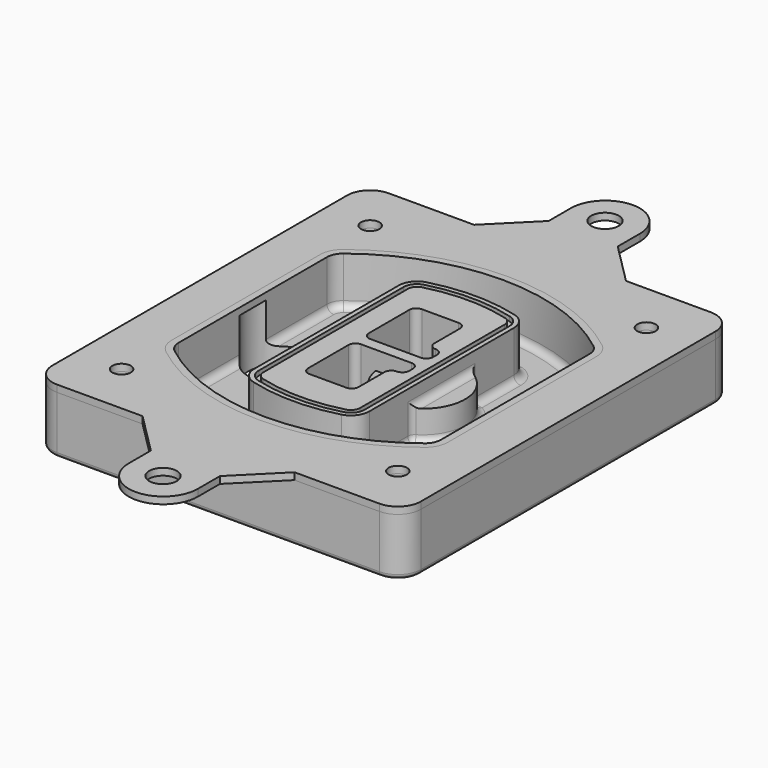
from build123d import *

# Parameters (mm, degrees)
F0_R      = 4
F1_DEPTH  = 25
F2_DEPTH  = 3
F3_DEPTH  = 18
F5_DEPTH  = 21
F6_DEPTH  = 2
F8_DEPTH  = 20
F9_DEPTH  = 16
F10_DEPTH = 25
F7_R      = 6
F7_R_2    = 4
F11_DEPTH = 6
F13_DEPTH = 9
F14_R     = 3
F15_R     = 2
F16_R     = 6
F16_R_2   = 4
F17_DEPTH = 3


with BuildPart() as f1:
    # F0 (on Top) → F1 (new body)
    with BuildSketch(Plane.XY):
        with BuildLine():
            ThreePointArc((-80, -80), (-77.0710678119, -87.0710678119), (-70, -90))
            Line((-70, -90), (70, -90))
            ThreePointArc((70, -90), (77.0710678119, -87.0710678119), (80, -80))
            Line((80, -80), (80, 80))
            ThreePointArc((80, 80), (77.0710678119, 87.0710678119), (70, 90))
            Line((70, 90), (-70, 90))
            ThreePointArc((-70, 90), (-77.0710678119, 87.0710678119), (-80, 80))
            Line((-80, 80), (-80, -80))
        make_face()
        with Locations((-60, -67.5)):
            Circle(F0_R, mode=Mode.SUBTRACT)
        with Locations((60, -67.5)):
            Circle(F0_R, mode=Mode.SUBTRACT)
        with Locations((-60, 67.5)):
            Circle(F0_R, mode=Mode.SUBTRACT)
        with BuildLine():
            ThreePointArc((-64, 40.2934422872), (-62.5820384798, 46.4328484224), (-58.6153846154, 51.3286200352))
            ThreePointArc((-58.6153846154, 51.3286200352), (0, 71.5), (58.6153846154, 51.3286200352))
            ThreePointArc((58.6153846154, 51.3286200352), (62.5820384798, 46.4328484224), (64, 40.2934422872))
            Line((64, 40.2934422872), (64, -40.2934422872))
            ThreePointArc((64, -40.2934422872), (62.5820384798, -46.4328484224), (58.6153846154, -51.3286200352))
            ThreePointArc((58.6153846154, -51.3286200352), (0, -71.5), (-58.6153846154, -51.3286200352))
            ThreePointArc((-58.6153846154, -51.3286200352), (-62.5820384798, -46.4328484224), (-64, -40.2934422872))
            Line((-64, -40.2934422872), (-64, 40.2934422872))
        make_face(mode=Mode.SUBTRACT)
        with Locations((60, 67.5)):
            Circle(F0_R, mode=Mode.SUBTRACT)
        with BuildLine():
            ThreePointArc((58.6153846154, 51.3286200352), (0, 71.5), (-58.6153846154, 51.3286200352))
            ThreePointArc((-58.6153846154, 51.3286200352), (-62.5820384798, 46.4328484224), (-64, 40.2934422872))
            Line((-64, 40.2934422872), (-64, -40.2934422872))
            ThreePointArc((-64, -40.2934422872), (-62.5820384798, -46.4328484224), (-58.6153846154, -51.3286200352))
            ThreePointArc((-58.6153846154, -51.3286200352), (0, -71.5), (58.6153846154, -51.3286200352))
            ThreePointArc((58.6153846154, -51.3286200352), (62.5820384798, -46.4328484224), (64, -40.2934422872))
            Line((64, -40.2934422872), (64, 40.2934422872))
            ThreePointArc((64, 40.2934422872), (62.5820384798, 46.4328484224), (58.6153846154, 51.3286200352))
        make_face()
        with BuildLine():
            Line((-60, -40.2934422872), (-60, 40.2934422872))
            ThreePointArc((-60, 40.2934422872), (-58.9871703427, 44.6787323838), (-56.1538461538, 48.1757121072))
            ThreePointArc((-56.1538461538, 48.1757121072), (0, 67.5), (56.1538461538, 48.1757121072))
            ThreePointArc((56.1538461538, 48.1757121072), (58.9871703427, 44.6787323838), (60, 40.2934422872))
            Line((60, 40.2934422872), (60, -40.2934422872))
            ThreePointArc((60, -40.2934422872), (58.9871703427, -44.6787323838), (56.1538461538, -48.1757121072))
            ThreePointArc((56.1538461538, -48.1757121072), (0, -67.5), (-56.1538461538, -48.1757121072))
            ThreePointArc((-56.1538461538, -48.1757121072), (-58.9871703427, -44.6787323838), (-60, -40.2934422872))
        make_face(mode=Mode.SUBTRACT)
        with BuildLine():
            ThreePointArc((-56.1538461538, 48.1757121072), (-58.9871703427, 44.6787323838), (-60, 40.2934422872))
            Line((-60, 40.2934422872), (-60, -40.2934422872))
            ThreePointArc((-60, -40.2934422872), (-58.9871703427, -44.6787323838), (-56.1538461538, -48.1757121072))
            ThreePointArc((-56.1538461538, -48.1757121072), (0, -67.5), (56.1538461538, -48.1757121072))
            ThreePointArc((56.1538461538, -48.1757121072), (58.9871703427, -44.6787323838), (60, -40.2934422872))
            Line((60, -40.2934422872), (60, 40.2934422872))
            ThreePointArc((60, 40.2934422872), (58.9871703427, 44.6787323838), (56.1538461538, 48.1757121072))
            ThreePointArc((56.1538461538, 48.1757121072), (0, 67.5), (-56.1538461538, 48.1757121072))
        make_face()
        with BuildLine():
            ThreePointArc((54.3076923077, 45.8110311612), (56.2910192399, 43.3631453548), (57, 40.2934422872))
            Line((57, 40.2934422872), (57, -40.2934422872))
            ThreePointArc((57, -40.2934422872), (56.2910192399, -43.3631453548), (54.3076923077, -45.8110311612))
            ThreePointArc((54.3076923077, -45.8110311612), (0, -64.5), (-54.3076923077, -45.8110311612))
            ThreePointArc((-54.3076923077, -45.8110311612), (-56.2910192399, -43.3631453548), (-57, -40.2934422872))
            Line((-57, -40.2934422872), (-57, 40.2934422872))
            ThreePointArc((-57, 40.2934422872), (-56.2910192399, 43.3631453548), (-54.3076923077, 45.8110311612))
            ThreePointArc((-54.3076923077, 45.8110311612), (0, 64.5), (54.3076923077, 45.8110311612))
        make_face(mode=Mode.SUBTRACT)
        with BuildLine():
            Line((57, -40.2934422872), (57, 40.2934422872))
            ThreePointArc((57, 40.2934422872), (56.2910192399, 43.3631453548), (54.3076923077, 45.8110311612))
            ThreePointArc((54.3076923077, 45.8110311612), (0, 64.5), (-54.3076923077, 45.8110311612))
            ThreePointArc((-54.3076923077, 45.8110311612), (-56.2910192399, 43.3631453548), (-57, 40.2934422872))
            Line((-57, 40.2934422872), (-57, -40.2934422872))
            ThreePointArc((-57, -40.2934422872), (-56.2910192399, -43.3631453548), (-54.3076923077, -45.8110311612))
            ThreePointArc((-54.3076923077, -45.8110311612), (0, -64.5), (54.3076923077, -45.8110311612))
            ThreePointArc((54.3076923077, -45.8110311612), (56.2910192399, -43.3631453548), (57, -40.2934422872))
        make_face()
    extrude(amount=-F1_DEPTH)

    # F0 (on Top) → F2 (join)
    with BuildSketch(Plane.XY):
        with BuildLine():
            ThreePointArc((-56.1538461538, 48.1757121072), (-58.9871703427, 44.6787323838), (-60, 40.2934422872))
            Line((-60, 40.2934422872), (-60, -40.2934422872))
            ThreePointArc((-60, -40.2934422872), (-58.9871703427, -44.6787323838), (-56.1538461538, -48.1757121072))
            ThreePointArc((-56.1538461538, -48.1757121072), (0, -67.5), (56.1538461538, -48.1757121072))
            ThreePointArc((56.1538461538, -48.1757121072), (58.9871703427, -44.6787323838), (60, -40.2934422872))
            Line((60, -40.2934422872), (60, 40.2934422872))
            ThreePointArc((60, 40.2934422872), (58.9871703427, 44.6787323838), (56.1538461538, 48.1757121072))
            ThreePointArc((56.1538461538, 48.1757121072), (0, 67.5), (-56.1538461538, 48.1757121072))
        make_face()
        with BuildLine():
            ThreePointArc((54.3076923077, 45.8110311612), (56.2910192399, 43.3631453548), (57, 40.2934422872))
            Line((57, 40.2934422872), (57, -40.2934422872))
            ThreePointArc((57, -40.2934422872), (56.2910192399, -43.3631453548), (54.3076923077, -45.8110311612))
            ThreePointArc((54.3076923077, -45.8110311612), (0, -64.5), (-54.3076923077, -45.8110311612))
            ThreePointArc((-54.3076923077, -45.8110311612), (-56.2910192399, -43.3631453548), (-57, -40.2934422872))
            Line((-57, -40.2934422872), (-57, 40.2934422872))
            ThreePointArc((-57, 40.2934422872), (-56.2910192399, 43.3631453548), (-54.3076923077, 45.8110311612))
            ThreePointArc((-54.3076923077, 45.8110311612), (0, 64.5), (54.3076923077, 45.8110311612))
        make_face(mode=Mode.SUBTRACT)
    extrude(amount=F2_DEPTH)

    # F0 (on Top) → F3 (cut)
    with BuildSketch(Plane.XY):
        with BuildLine():
            Line((57, -40.2934422872), (57, 40.2934422872))
            ThreePointArc((57, 40.2934422872), (56.2910192399, 43.3631453548), (54.3076923077, 45.8110311612))
            ThreePointArc((54.3076923077, 45.8110311612), (0, 64.5), (-54.3076923077, 45.8110311612))
            ThreePointArc((-54.3076923077, 45.8110311612), (-56.2910192399, 43.3631453548), (-57, 40.2934422872))
            Line((-57, 40.2934422872), (-57, -40.2934422872))
            ThreePointArc((-57, -40.2934422872), (-56.2910192399, -43.3631453548), (-54.3076923077, -45.8110311612))
            ThreePointArc((-54.3076923077, -45.8110311612), (0, -64.5), (54.3076923077, -45.8110311612))
            ThreePointArc((54.3076923077, -45.8110311612), (56.2910192399, -43.3631453548), (57, -40.2934422872))
        make_face()
    extrude(amount=-F3_DEPTH, mode=Mode.SUBTRACT)

    # F4 (on face) → F5 (join, through all)
    with BuildSketch(Plane.XY.offset(3)):
        with BuildLine():
            ThreePointArc((-25, -39.2465276821), (-23.3511545998, -44.1109737193), (-19.0842911877, -46.9702398883))
            ThreePointArc((-19.0842911877, -46.9702398883), (0, -49.5), (19.0842911877, -46.9702398883))
            ThreePointArc((19.0842911877, -46.9702398883), (23.3511545998, -44.1109737193), (25, -39.2465276821))
            Line((25, -39.2465276821), (25, 39.2465276821))
            ThreePointArc((25, 39.2465276821), (23.3511545998, 44.1109737193), (19.0842911877, 46.9702398883))
            ThreePointArc((19.0842911877, 46.9702398883), (0, 49.5), (-19.0842911877, 46.9702398883))
            ThreePointArc((-19.0842911877, 46.9702398883), (-23.3511545998, 44.1109737193), (-25, 39.2465276821))
            Line((-25, 39.2465276821), (-25, -39.2465276821))
        make_face()
        with BuildLine():
            ThreePointArc((18.5632183908, 45.0393118368), (21.7633659499, 42.89486221), (23, 39.2465276821))
            Line((23, 39.2465276821), (23, -39.2465276821))
            ThreePointArc((23, -39.2465276821), (21.7633659499, -42.89486221), (18.5632183908, -45.0393118368))
            ThreePointArc((18.5632183908, -45.0393118368), (0, -47.5), (-18.5632183908, -45.0393118368))
            ThreePointArc((-18.5632183908, -45.0393118368), (-21.7633659499, -42.89486221), (-23, -39.2465276821))
            Line((-23, -39.2465276821), (-23, 39.2465276821))
            ThreePointArc((-23, 39.2465276821), (-21.7633659499, 42.89486221), (-18.5632183908, 45.0393118368))
            ThreePointArc((-18.5632183908, 45.0393118368), (0, 47.5), (18.5632183908, 45.0393118368))
        make_face(mode=Mode.SUBTRACT)
        with BuildLine():
            Line((23, -39.2465276821), (23, 39.2465276821))
            ThreePointArc((23, 39.2465276821), (21.7633659499, 42.89486221), (18.5632183908, 45.0393118368))
            ThreePointArc((18.5632183908, 45.0393118368), (0, 47.5), (-18.5632183908, 45.0393118368))
            ThreePointArc((-18.5632183908, 45.0393118368), (-21.7633659499, 42.89486221), (-23, 39.2465276821))
            Line((-23, 39.2465276821), (-23, -39.2465276821))
            ThreePointArc((-23, -39.2465276821), (-21.7633659499, -42.89486221), (-18.5632183908, -45.0393118368))
            ThreePointArc((-18.5632183908, -45.0393118368), (0, -47.5), (18.5632183908, -45.0393118368))
            ThreePointArc((18.5632183908, -45.0393118368), (21.7633659499, -42.89486221), (23, -39.2465276821))
        make_face()
        with BuildLine():
            ThreePointArc((18.0421455939, 43.1083837852), (20.1755772999, 41.6787507007), (21, 39.2465276821))
            Line((21, 39.2465276821), (21, -39.2465276821))
            ThreePointArc((21, -39.2465276821), (20.1755772999, -41.6787507007), (18.0421455939, -43.1083837852))
            ThreePointArc((18.0421455939, -43.1083837852), (0, -45.5), (-18.0421455939, -43.1083837852))
            ThreePointArc((-18.0421455939, -43.1083837852), (-20.1755772999, -41.6787507007), (-21, -39.2465276821))
            Line((-21, -39.2465276821), (-21, 39.2465276821))
            ThreePointArc((-21, 39.2465276821), (-20.1755772999, 41.6787507007), (-18.0421455939, 43.1083837852))
            ThreePointArc((-18.0421455939, 43.1083837852), (0, 45.5), (18.0421455939, 43.1083837852))
        make_face(mode=Mode.SUBTRACT)
        with BuildLine():
            Line((21, -39.2465276821), (21, 39.2465276821))
            ThreePointArc((21, 39.2465276821), (20.1755772999, 41.6787507007), (18.0421455939, 43.1083837852))
            ThreePointArc((18.0421455939, 43.1083837852), (0, 45.5), (-18.0421455939, 43.1083837852))
            ThreePointArc((-18.0421455939, 43.1083837852), (-20.1755772999, 41.6787507007), (-21, 39.2465276821))
            Line((-21, 39.2465276821), (-21, -39.2465276821))
            ThreePointArc((-21, -39.2465276821), (-20.1755772999, -41.6787507007), (-18.0421455939, -43.1083837852))
            ThreePointArc((-18.0421455939, -43.1083837852), (0, -45.5), (18.0421455939, -43.1083837852))
            ThreePointArc((18.0421455939, -43.1083837852), (20.1755772999, -41.6787507007), (21, -39.2465276821))
        make_face()
        with BuildLine():
            Line((-8, -2.5), (14, -2.5))
            ThreePointArc((14, -2.5), (16.1213203436, -3.3786796564), (17, -5.5))
            Line((17, -5.5), (17, -7.5))
            ThreePointArc((17, -7.5), (16.1213203436, -9.6213203436), (14, -10.5))
            ThreePointArc((14, -10.5), (11.8786796564, -11.3786796564), (11, -13.5))
            Line((11, -13.5), (11, -27.5))
            ThreePointArc((11, -27.5), (10.1213203436, -29.6213203436), (8, -30.5))
            Line((8, -30.5), (-8, -30.5))
            ThreePointArc((-8, -30.5), (-10.1213203436, -29.6213203436), (-11, -27.5))
            Line((-11, -27.5), (-11, -5.5))
            ThreePointArc((-11, -5.5), (-10.1213203436, -3.3786796564), (-8, -2.5))
        make_face(mode=Mode.SUBTRACT)
        with BuildLine():
            ThreePointArc((-8, 2.5), (-10.1213203436, 3.3786796564), (-11, 5.5))
            Line((-11, 5.5), (-11, 27.5))
            ThreePointArc((-11, 27.5), (-10.1213203436, 29.6213203436), (-8, 30.5))
            Line((-8, 30.5), (8, 30.5))
            ThreePointArc((8, 30.5), (10.1213203436, 29.6213203436), (11, 27.5))
            Line((11, 27.5), (11, 13.5))
            ThreePointArc((11, 13.5), (11.8786796564, 11.3786796564), (14, 10.5))
            ThreePointArc((14, 10.5), (16.1213203436, 9.6213203436), (17, 7.5))
            Line((17, 7.5), (17, 5.5))
            ThreePointArc((17, 5.5), (16.1213203436, 3.3786796564), (14, 2.5))
            Line((14, 2.5), (-8, 2.5))
        make_face(mode=Mode.SUBTRACT)
    extrude(amount=-F5_DEPTH)

    # F4 (on face) → F6 (cut)
    with BuildSketch(Plane.XY.offset(3)):
        with BuildLine():
            Line((23, -39.2465276821), (23, 39.2465276821))
            ThreePointArc((23, 39.2465276821), (21.7633659499, 42.89486221), (18.5632183908, 45.0393118368))
            ThreePointArc((18.5632183908, 45.0393118368), (0, 47.5), (-18.5632183908, 45.0393118368))
            ThreePointArc((-18.5632183908, 45.0393118368), (-21.7633659499, 42.89486221), (-23, 39.2465276821))
            Line((-23, 39.2465276821), (-23, -39.2465276821))
            ThreePointArc((-23, -39.2465276821), (-21.7633659499, -42.89486221), (-18.5632183908, -45.0393118368))
            ThreePointArc((-18.5632183908, -45.0393118368), (0, -47.5), (18.5632183908, -45.0393118368))
            ThreePointArc((18.5632183908, -45.0393118368), (21.7633659499, -42.89486221), (23, -39.2465276821))
        make_face()
        with BuildLine():
            ThreePointArc((18.0421455939, 43.1083837852), (20.1755772999, 41.6787507007), (21, 39.2465276821))
            Line((21, 39.2465276821), (21, -39.2465276821))
            ThreePointArc((21, -39.2465276821), (20.1755772999, -41.6787507007), (18.0421455939, -43.1083837852))
            ThreePointArc((18.0421455939, -43.1083837852), (0, -45.5), (-18.0421455939, -43.1083837852))
            ThreePointArc((-18.0421455939, -43.1083837852), (-20.1755772999, -41.6787507007), (-21, -39.2465276821))
            Line((-21, -39.2465276821), (-21, 39.2465276821))
            ThreePointArc((-21, 39.2465276821), (-20.1755772999, 41.6787507007), (-18.0421455939, 43.1083837852))
            ThreePointArc((-18.0421455939, 43.1083837852), (0, 45.5), (18.0421455939, 43.1083837852))
        make_face(mode=Mode.SUBTRACT)
    extrude(amount=-F6_DEPTH, mode=Mode.SUBTRACT)

    # F7 (on face) → F8 (join)
    with BuildSketch(Plane(origin=(0, 0, -25), x_dir=(1, 0, 0), z_dir=(0, 0, -1))):
        with BuildLine():
            ThreePointArc((3.28842436, 0), (16.7567035675, 13.4682792075), (30.224982775, 0))
            Line((30.224982775, 0), (35.224982775, 0))
            ThreePointArc((35.224982775, 0), (16.7567035675, 18.4682792075), (-1.71157564, 0))
            Line((-1.71157564, 0), (3.28842436, 0))
        make_face()
        with BuildLine():
            Line((3.28842436, 0), (30.224982775, 0))
            ThreePointArc((30.224982775, 0), (16.7567035675, 13.4682792075), (3.28842436, 0))
        make_face()
        with BuildLine():
            ThreePointArc((3.28842436, 0), (16.7567035675, -13.4682792075), (30.224982775, 0))
            Line((30.224982775, 0), (3.28842436, 0))
        make_face()
        with BuildLine():
            Line((35.224982775, 0), (30.224982775, 0))
            ThreePointArc((30.224982775, 0), (16.7567035675, -13.4682792075), (3.28842436, 0))
            Line((3.28842436, 0), (-1.71157564, 0))
            ThreePointArc((-1.71157564, 0), (16.7567035675, -18.4682792075), (35.224982775, 0))
        make_face()
    extrude(amount=-F8_DEPTH)

    # F7 (on face) → F9 (cut)
    with BuildSketch(Plane(origin=(0, 0, -25), x_dir=(1, 0, 0), z_dir=(0, 0, -1))):
        with BuildLine():
            Line((3.28842436, 0), (30.224982775, 0))
            ThreePointArc((30.224982775, 0), (16.7567035675, 13.4682792075), (3.28842436, 0))
        make_face()
        with BuildLine():
            ThreePointArc((3.28842436, 0), (16.7567035675, -13.4682792075), (30.224982775, 0))
            Line((30.224982775, 0), (3.28842436, 0))
        make_face()
    extrude(amount=-F9_DEPTH, mode=Mode.SUBTRACT)

    # F7 (on face) → F10 (cut)
    with BuildSketch(Plane(origin=(0, 0, -25), x_dir=(1, 0, 0), z_dir=(0, 0, -1))):
        with BuildLine():
            Line((-59.0318229325, 0), (-32.0952645175, 0))
            ThreePointArc((-32.0952645175, 0), (-45.563543725, 13.4682792075), (-59.0318229325, 0))
        make_face()
        with BuildLine():
            ThreePointArc((-59.0318229325, 0), (-45.563543725, -13.4682792075), (-32.0952645175, 0))
            Line((-32.0952645175, 0), (-59.0318229325, 0))
        make_face()
    extrude(amount=-F10_DEPTH, mode=Mode.SUBTRACT)

    # F7 (on face) → F11 (cut)
    with BuildSketch(Plane(origin=(0, 0, -25), x_dir=(1, 0, 0), z_dir=(0, 0, -1))):
        with Locations((60, -67.5)):
            Circle(F7_R)
        with Locations((60, -67.5)):
            Circle(F7_R_2, mode=Mode.SUBTRACT)
        with Locations((-60, -67.5)):
            Circle(F7_R)
        with Locations((-60, -67.5)):
            Circle(F7_R_2, mode=Mode.SUBTRACT)
        with Locations((-60, 67.5)):
            Circle(F7_R)
        with Locations((-60, 67.5)):
            Circle(F7_R_2, mode=Mode.SUBTRACT)
        with Locations((60, 67.5)):
            Circle(F7_R)
        with Locations((60, 67.5)):
            Circle(F7_R_2, mode=Mode.SUBTRACT)
    extrude(amount=-F11_DEPTH, mode=Mode.SUBTRACT)

    # F12 (on face) → F13 (cut, through all)
    with BuildSketch(Plane(origin=(0, 0, -9), x_dir=(1, 0, 0), z_dir=(0, 0, -1))):
        with BuildLine():
            Line((11, 13.5), (11, 17.5481537753))
            ThreePointArc((11, 17.5481537753), (2.5696536419, 11.8239143813), (-1.5415842455, 2.5))
            Line((-1.5415842455, 2.5), (3.5224848595, 2.5))
            ThreePointArc((3.5224848595, 2.5), (6.1857188154, 8.3455872281), (11.2536447004, 12.2927168648))
            ThreePointArc((11.2536447004, 12.2927168648), (11.0640958889, 12.8831798879), (11, 13.5))
        make_face()
        with BuildLine():
            ThreePointArc((11.2536447004, -12.2927168648), (6.1857188154, -8.3455872281), (3.5224848595, -2.5))
            Line((3.5224848595, -2.5), (-1.5415842455, -2.5))
            ThreePointArc((-1.5415842455, -2.5), (2.5696536419, -11.8239143813), (11, -17.5481537753))
            Line((11, -17.5481537753), (11, -13.5))
            ThreePointArc((11, -13.5), (11.0640958889, -12.8831798879), (11.2536447004, -12.2927168648))
        make_face()
        with BuildLine():
            ThreePointArc((11.2536447004, 12.2927168648), (6.1857188154, 8.3455872281), (3.5224848595, 2.5))
            Line((3.5224848595, 2.5), (14, 2.5))
            ThreePointArc((14, 2.5), (16.1213203436, 3.3786796564), (17, 5.5))
            Line((17, 5.5), (17, 7.5))
            ThreePointArc((17, 7.5), (16.1213203436, 9.6213203436), (14, 10.5))
            ThreePointArc((14, 10.5), (12.3601599782, 10.9878446101), (11.2536447004, 12.2927168648))
        make_face()
        with BuildLine():
            Line((14, -2.5), (3.5224848595, -2.5))
            ThreePointArc((3.5224848595, -2.5), (6.1857188154, -8.3455872281), (11.2536447004, -12.2927168648))
            ThreePointArc((11.2536447004, -12.2927168648), (12.3601599782, -10.9878446101), (14, -10.5))
            ThreePointArc((14, -10.5), (16.1213203436, -9.6213203436), (17, -7.5))
            Line((17, -7.5), (17, -5.5))
            ThreePointArc((17, -5.5), (16.1213203436, -3.3786796564), (14, -2.5))
        make_face()
    extrude(amount=F13_DEPTH, mode=Mode.SUBTRACT)

    # F14
    f14_edges = [f1.edges().sort_by_distance(p)[0] for p in [
        (-57, -23.703476, -18),
        (-57, 23.703476, -18),
        (25, 0, -5),
        (25, 16.526506, -11.5),
        (25, -16.526506, -11.5),
        (25, -27.886517, -18),
        (35.224983, 0, -18),
    ]]
    fillet(f14_edges, radius=F14_R)

    # F15
    f15_edges = [f1.edges().sort_by_distance(p)[0] for p in [
        (0, -90, -25),
    ]]
    fillet(f15_edges, radius=F15_R)


with BuildPart() as f17:
    # F16 (on face) → F17 (new body, through all)
    with BuildSketch(Plane.XY):
        with BuildLine():
            Line((-14.8738344499, 108), (-32.8738344499, 90))
            Line((-32.8738344499, 90), (33.1261655501, 90))
            Line((33.1261655501, 90), (15.1261655501, 108))
            Line((15.1261655501, 108), (15.1261655501, 120))
            ThreePointArc((15.1261655501, 120), (0.1261655501, 135), (-14.8738344499, 120))
            Line((-14.8738344499, 120), (-14.8738344499, 108))
        make_face()
        with Locations((0, 120)):
            Circle(F16_R, mode=Mode.SUBTRACT)
        with BuildLine():
            Line((33.1261655501, -90), (-32.8738344499, -90))
            Line((-32.8738344499, -90), (-14.8738344499, -108))
            Line((-14.8738344499, -108), (-14.8738344499, -120))
            ThreePointArc((-14.8738344499, -120), (0.1261655501, -135), (15.1261655501, -120))
            Line((15.1261655501, -120), (15.1261655501, -108))
            Line((15.1261655501, -108), (33.1261655501, -90))
        make_face()
        with Locations((0, -120)):
            Circle(F16_R, mode=Mode.SUBTRACT)
        with BuildLine():
            Line((33.1261655501, 90), (-32.8738344499, 90))
            Line((-32.8738344499, 90), (-70, 90))
            ThreePointArc((-70, 90), (-77.0710678119, 87.0710678119), (-80, 80))
            Line((-80, 80), (-80, -80))
            ThreePointArc((-80, -80), (-77.0710678119, -87.0710678119), (-70, -90))
            Line((-70, -90), (-32.8738344499, -90))
            Line((-32.8738344499, -90), (33.1261655501, -90))
            Line((33.1261655501, -90), (70, -90))
            ThreePointArc((70, -90), (77.0710678119, -87.0710678119), (80, -80))
            Line((80, -80), (80, 80))
            ThreePointArc((80, 80), (77.0710678119, 87.0710678119), (70, 90))
            Line((70, 90), (33.1261655501, 90))
        make_face()
        with Locations((-60, -67.5)):
            Circle(F16_R_2, mode=Mode.SUBTRACT)
        with Locations((60, -67.5)):
            Circle(F16_R_2, mode=Mode.SUBTRACT)
        with Locations((-60, 67.5)):
            Circle(F16_R_2, mode=Mode.SUBTRACT)
        with BuildLine():
            ThreePointArc((-60, 40.2934422872), (-58.9871703427, 44.6787323838), (-56.1538461538, 48.1757121072))
            ThreePointArc((-56.1538461538, 48.1757121072), (0, 67.5), (56.1538461538, 48.1757121072))
            ThreePointArc((56.1538461538, 48.1757121072), (58.9871703427, 44.6787323838), (60, 40.2934422872))
            Line((60, 40.2934422872), (60, -40.2934422872))
            ThreePointArc((60, -40.2934422872), (58.9871703427, -44.6787323838), (56.1538461538, -48.1757121072))
            ThreePointArc((56.1538461538, -48.1757121072), (0, -67.5), (-56.1538461538, -48.1757121072))
            ThreePointArc((-56.1538461538, -48.1757121072), (-58.9871703427, -44.6787323838), (-60, -40.2934422872))
            Line((-60, -40.2934422872), (-60, 40.2934422872))
        make_face(mode=Mode.SUBTRACT)
        with Locations((60, 67.5)):
            Circle(F16_R_2, mode=Mode.SUBTRACT)
    extrude(amount=F17_DEPTH)


solid = Compound([f1.part, f17.part])
